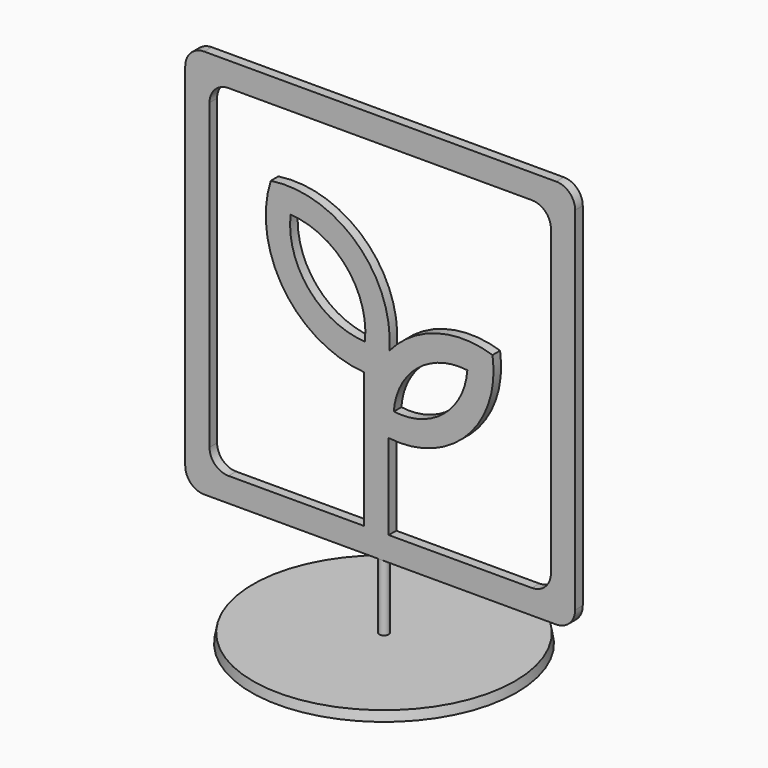
from build123d import *

# Parameters (mm, degrees)
F2_DEPTH = 3.175
F3_R     = 1.5875
F4_DEPTH = 25.4
F5_R     = 44.45
F6_DEPTH = 3.175
F6_TAPER = 10


# Not quite as in the source:
# - a feature of the source that left no trace in its solid (it failed there, or was rolled back) is left out


with BuildPart() as f2:
    # F1 (on Front) → F2 (new body)
    with BuildSketch(Plane.XZ):
        with BuildLine():
            Line((58.928, 65.278), (-58.928, 65.278))
            ThreePointArc((-58.928, 65.278), (-63.4181280605, 63.4181280605), (-65.278, 58.928))
            Line((-65.278, 58.928), (-65.278, -58.928))
            ThreePointArc((-65.278, -58.928), (-63.4181280605, -63.4181280605), (-58.928, -65.278))
            Line((-58.928, -65.278), (58.928, -65.278))
            ThreePointArc((58.928, -65.278), (63.4181280605, -63.4181280605), (65.278, -58.928))
            Line((65.278, -58.928), (65.278, 58.928))
            ThreePointArc((65.278, 58.928), (63.4181280605, 63.4181280605), (58.928, 65.278))
        make_face()
        with BuildLine():
            ThreePointArc((29.1683860123, 0), (21.2359008795, -15.4304684341), (4.5518055526, -20.1912078303))
            ThreePointArc((4.5518055526, -20.1912078303), (12.5076591177, -4.7892295638), (29.1683860123, 0))
        make_face(mode=Mode.SUBTRACT)
        with BuildLine():
            ThreePointArc((-30.0225467432, 26.633475086), (-11.3001914874, 17.269662026), (-5.1093608776, -2.7273676961))
            ThreePointArc((-5.1093608776, -2.7273676961), (-23.8921161087, 6.5851949341), (-30.0225467432, 26.633475086))
        make_face(mode=Mode.SUBTRACT)
        with BuildLine():
            Line((-5.3865113296, -11.8381703437), (-5.3865113296, -57.15))
            Line((-5.3865113296, -57.15), (-50.8, -57.15))
            ThreePointArc((-50.8, -57.15), (-55.2901280605, -55.2901280605), (-57.15, -50.8))
            Line((-57.15, -50.8), (-57.15, 50.8))
            ThreePointArc((-57.15, 50.8), (-55.2901280605, 55.2901280605), (-50.8, 57.15))
            Line((-50.8, 57.15), (50.8, 57.15))
            ThreePointArc((50.8, 57.15), (55.2901280605, 55.2901280605), (57.15, 50.8))
            Line((57.15, 50.8), (57.15, -50.8))
            ThreePointArc((57.15, -50.8), (55.2901280605, -55.2901280605), (50.8, -57.15))
            Line((50.8, -57.15), (2.8426104691, -57.15))
            Line((2.8426104691, -57.15), (2.8426104691, -28.5558674872))
            ThreePointArc((2.8426104691, -28.5558674872), (29.0723668952, -19.260680993), (37.6052677218, 7.2268673576))
            ThreePointArc((37.6052677218, 7.2268673576), (18.8257654598, 7.524261984), (3.0884773301, -2.7273676961))
            ThreePointArc((3.0884773301, -2.7273676961), (-7.830876963, 25.422268659), (-36.6427004337, 34.4507321715))
            ThreePointArc((-36.6427004337, 34.4507321715), (-32.213387286, 3.7443986853), (-5.3865113296, -11.8381703437))
        make_face(mode=Mode.SUBTRACT)
    extrude(amount=F2_DEPTH)

    # F3 (on face) → F4 (join)
    with BuildSketch(Plane(origin=(0, 0, -65.278), x_dir=(1, 0, 0), z_dir=(0, 0, -1))):
        with Locations((0, 1.5875)):
            Circle(F3_R)
    extrude(amount=F4_DEPTH)

    # F5 (on face) → F6 (join)
    with BuildSketch(Plane(origin=(0, 0, -90.678), x_dir=(1, 0, 0), z_dir=(0, 0, -1))):
        with Locations((0, 1.5875)):
            Circle(F5_R)
    extrude(amount=-F6_DEPTH, taper=F6_TAPER)


solid = f2.part
